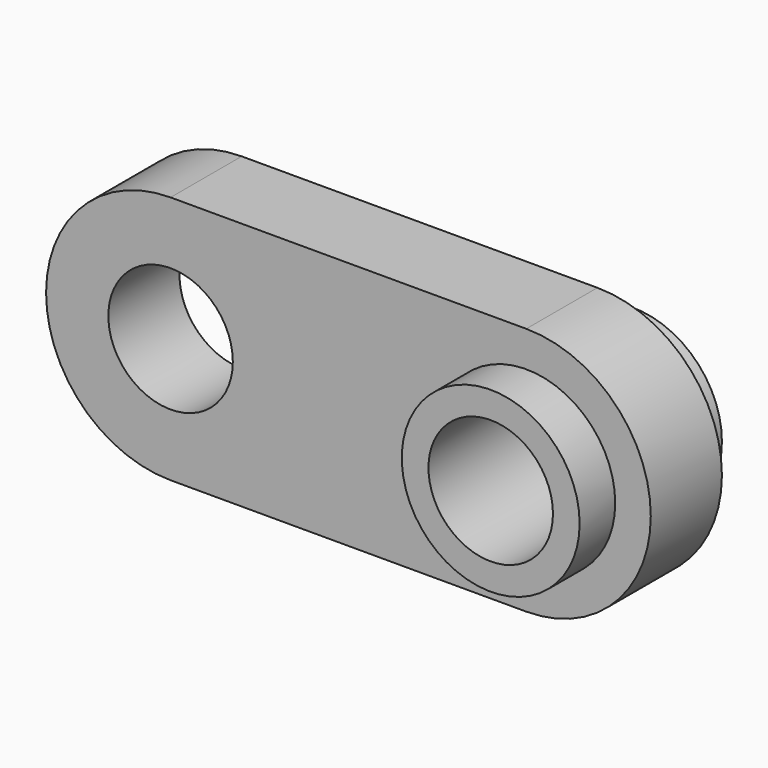
from build123d import *

# Parameters (mm, degrees)
F0_R     = 35
F1_DEPTH = 25
F2_R     = 50
F2_R_2   = 35
F3_DEPTH = 25


# Not quite as in the source:
# - a pattern or mirror of a feature is missing from the dataset's text; its kind, count and spacing are read off the source's solid


with BuildPart() as f1:
    # F0 (on Front) → F1 (new body, symmetric)
    with BuildSketch(Plane.XZ):
        with BuildLine():
            Line((100, 70), (-100, 70))
            ThreePointArc((-100, 70), (-170, 0), (-100, -70))
            Line((-100, -70), (100, -70))
            ThreePointArc((100, -70), (170, 0), (100, 70))
        make_face()
        with Locations((-100, 0)):
            Circle(F0_R, mode=Mode.SUBTRACT)
        with Locations((100, 0)):
            Circle(F0_R, mode=Mode.SUBTRACT)
    extrude(amount=F1_DEPTH, both=True)

    # F2 (on face) → F3 (join)
    with BuildSketch(Plane.XZ.offset(25)):
        with Locations((100, 0)):
            Circle(F2_R)
        with Locations((100, 0)):
            Circle(F2_R_2, mode=Mode.SUBTRACT)
    f3 = extrude(amount=F3_DEPTH)

    # F3_copies: F3 across plane
    add(f3.mirror(Plane.ZX))


solid = f1.part
